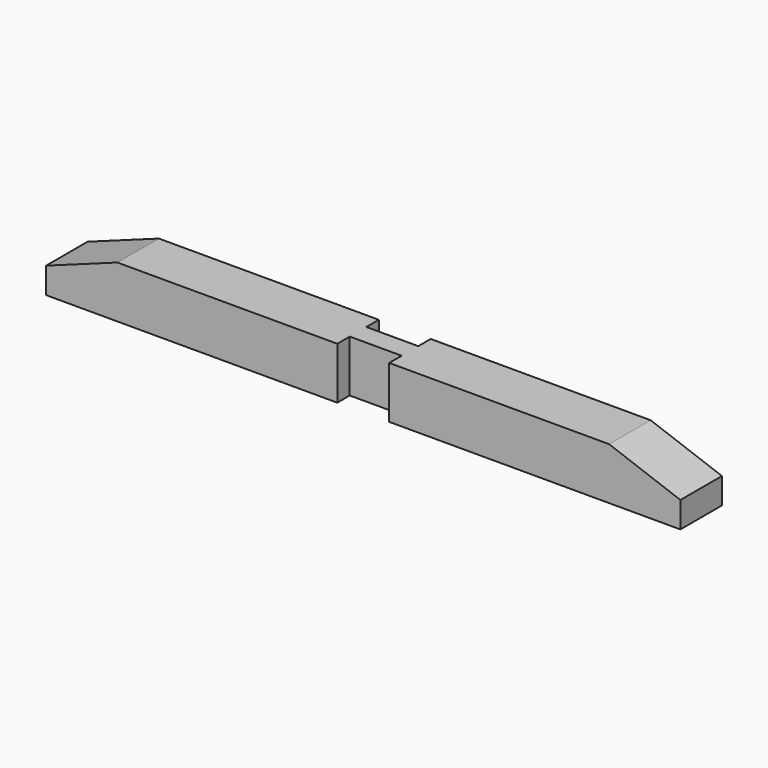
from build123d import *

# Parameters (mm, degrees)
F0_W     = 45
F0_H     = 45
F1_DEPTH = 275
F2_W     = 45
F2_H     = 13.5
F3_DEPTH = 45.001
F5_DEPTH = 45.001


# Not quite as in the source:
# - a pattern or mirror of a feature is missing from the dataset's text; its kind, count and spacing are read off the source's solid


with BuildPart() as f1:
    # F0 (on Right) → F1 (new body, symmetric)
    with BuildSketch(Plane.YZ):
        Rectangle(F0_W, F0_H)
    extrude(amount=F1_DEPTH, both=True)

    # F2 (on face) → F3 (cut, through all)
    with BuildSketch(Plane.XY.offset(22.5)):
        with Locations((0, 15.75)):
            Rectangle(F2_W, F2_H)
        with Locations((0, -15.75)):
            Rectangle(F2_W, F2_H)
    extrude(amount=-F3_DEPTH, mode=Mode.SUBTRACT)

    # F4 (on face) → F5 (cut, through all)
    with BuildSketch(Plane.XZ.offset(22.5)):
        Polygon((275, 22.5), (213.1817580623, 22.5), (275, 0), align=None)
    f5 = extrude(amount=-F5_DEPTH, mode=Mode.SUBTRACT)

    # F5_copies: F5 across plane
    add(f5.mirror(Plane(origin=(0, 0, 0), x_dir=(0, 0, -1), z_dir=(-1, 0, 0))), mode=Mode.SUBTRACT)


solid = f1.part
